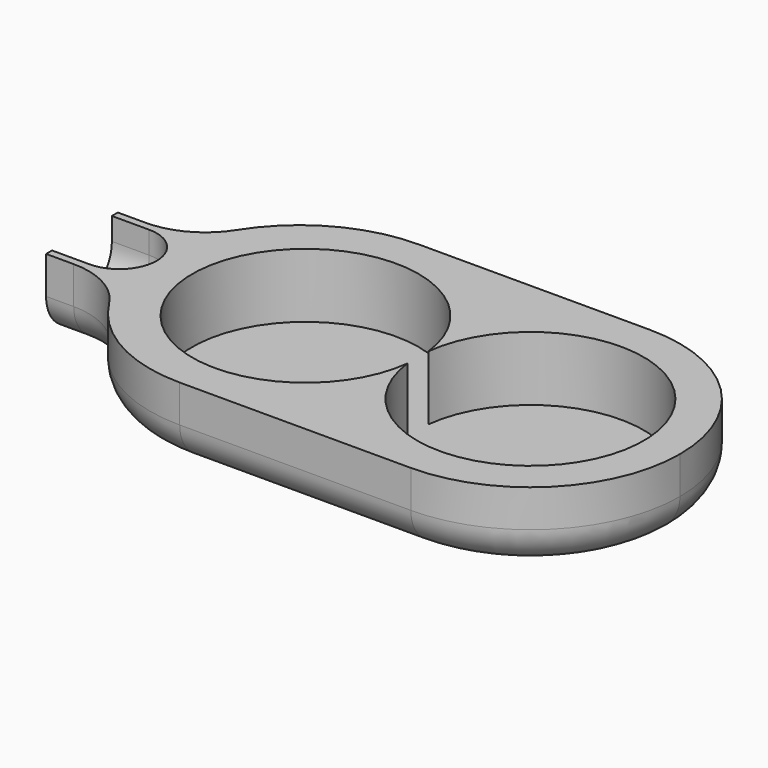
from build123d import *

# Parameters (mm, degrees)
F1_DEPTH    = 1
F2_R        = 1.515
F3_DEPTH    = 0.86
F4_R        = 1.515
F5_DEPTH    = 0.86
F6_DEPTH    = 0.6
F8_DEPTH    = 0.8
F9_T1_DEPTH = 10.5393920142
F9_T3_DEPTH = 11
F10_R       = 1
F11_R       = 0.49999
F12_R       = 0.5


# Not quite as in the source:
# - a fillet or chamfer that OpenCascade refuses, or shapes differently, is made with other operations: its cross-section is extruded or revolved along the edge and cut away or added
# - a fillet or chamfer is up to 0.001 mm smaller than in the source, because OpenCascade refuses the exact size


with BuildPart() as f1:
    # F0 (on Top) → F1 (new body)
    with BuildSketch(Plane.XY):
        Polygon((0, 1.4), (0, 0), (7, 0), (7, 4), (0, 4), (0, 2.6), (0, 2), align=None)
        Polygon((-1, 1.4), (0, 1.4), (0, 2), (0, 2.6), (-1, 2.6), align=None)
    extrude(amount=F1_DEPTH)

    # F2 (on face) → F3 (cut)
    with BuildSketch(Plane.XY.offset(1)):
        with Locations((5, 2)):
            Circle(F2_R)
    extrude(amount=-F3_DEPTH, mode=Mode.SUBTRACT)

    # F4 (on face) → F5 (cut)
    with BuildSketch(Plane.XY.offset(1)):
        with Locations((1.99, 2)):
            Circle(F4_R)
    extrude(amount=-F5_DEPTH, mode=Mode.SUBTRACT)

    # F4 (on face) → F6 (cut)
    with BuildSketch(Plane.XY.offset(1)):
        with Locations((1.99, 2)):
            Circle(F4_R)
    extrude(amount=-F6_DEPTH, mode=Mode.SUBTRACT)

    # F7 (on face) → F8 (cut)
    with BuildSketch(Plane.XY.offset(1)):
        Polygon((-1, 2.5), (-1, 2), (-1, 1.5), (0, 1.5), (0, 2.5), align=None)
    extrude(amount=-F8_DEPTH, mode=Mode.SUBTRACT)

    # F9: fillet of radius 2 on 4 edges, made by hand

    # F9_s2 → F9_t1 (cut)
    with BuildSketch(Plane.XY.offset(-4.7696960071)):
        with BuildLine():
            ThreePointArc((1.9078784028, 4), (0.7246624462, 3.6124515497), (0, 2.6))
            Line((0, 2.6), (-0.0381575681, 2.612))
            ThreePointArc((-0.0381575681, 2.612), (-0.04, 3.3), (-0.04, 4))
            Line((-0.04, 4), (0, 4.04))
            Line((0, 4.04), (1.9078784028, 4.04))
            Line((1.9078784028, 4.04), (1.9078784028, 4))
        make_face()
        with BuildLine():
            ThreePointArc((0, 1.4), (0.7246624462, 0.3875484503), (1.9078784028, 0))
            Line((1.9078784028, 0), (1.9078784028, -0.04))
            Line((1.9078784028, -0.04), (0, -0.04))
            Line((0, -0.04), (-0.04, 0))
            ThreePointArc((-0.04, 0), (-0.04, 0.7), (-0.0381575681, 1.388))
            Line((-0.0381575681, 1.388), (0, 1.4))
        make_face()
    extrude(amount=F9_T1_DEPTH, mode=Mode.SUBTRACT)

    # F9_s4 → F9_t3 (cut)
    with BuildSketch(Plane.XY.offset(-5)):
        with BuildLine():
            ThreePointArc((7, 2), (6.4142135624, 3.4142135624), (5, 4))
            Line((5, 4), (5, 4.04))
            Line((5, 4.04), (7.04, 4.04))
            Line((7.04, 4.04), (7.04, 2))
            Line((7.04, 2), (7, 2))
        make_face()
        with BuildLine():
            ThreePointArc((5, 0), (6.4142135624, 0.5857864376), (7, 2))
            Line((7, 2), (7.04, 2))
            Line((7.04, 2), (7.04, -0.04))
            Line((7.04, -0.04), (5, -0.04))
            Line((5, -0.04), (5, 0))
        make_face()
    extrude(amount=F9_T3_DEPTH, mode=Mode.SUBTRACT)

    # F10
    f10_edges = [f1.edges().sort_by_distance(p)[0] for p in [
        (0, 1.4, 0.5),
        (0, 2.6, 0.5),
    ]]
    fillet(f10_edges, radius=F10_R)

    # F11 (radius 0.5 in the source; OpenCascade refuses exactly that, so slightly less here)
    f11_edges = [f1.edges().sort_by_distance(p)[0] for p in [
        (-0.5, 2.5, 0.2),
        (-0.5, 1.5, 0.2),
        (0, 1.5, 0.6),
        (0, 2.5, 0.6),
        (0, 2, 0.2),
    ]]
    fillet(f11_edges, radius=F11_R)

    # F12
    f12_edges = [f1.edges().sort_by_distance(p)[0] for p in [
        (3.453939, 0, 0),
        (6.414214, 0.585786, 0),
    ]]
    fillet(f12_edges, radius=F12_R)


solid = f1.part
